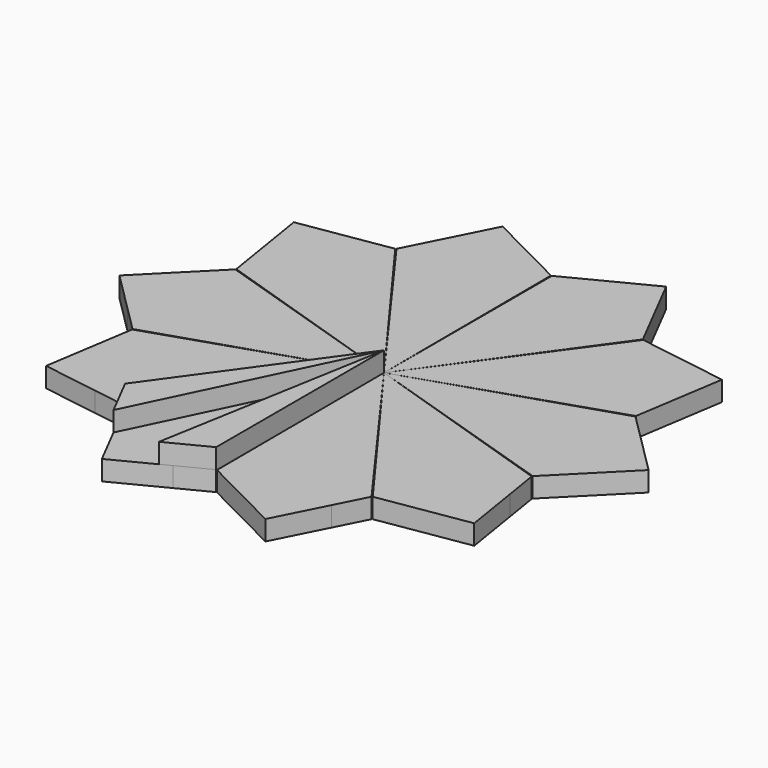
from build123d import *

# Parameters (mm, degrees)
F1_DEPTH = 10
F3_DEPTH = 10
F4_COUNT = 10


# Not quite as in the source:
# - a feature names something its author has since deleted; it is built from what else it names


with BuildPart() as f1:
    # F0 (on Top) → F1 (new body)
    with BuildSketch(Plane.XY):
        Polygon((-305.3184055859, -77.3749127087), (-289.8050833034, 36.5739215625), (-343.7715783939, -64.9771365691), (-330.7438800597, -90.4026110429), align=None)
        Polygon((-343.7715783939, -64.9771365691), (-289.8050833034, 36.5739215625), (-351.7204126651, -49.4638142865), align=None)
        Polygon((-289.8050833034, -69.4260784375), (-289.8050833034, 36.5739215625), (-305.3184055859, -77.3749127087), align=None)
    extrude(amount=F1_DEPTH)


with BuildPart() as f3:
    # F2 (on face) → F3 (new body)
    with BuildSketch(Plane.XY.offset(10)):
        Polygon((-289.8050833034, -69.4260784375), (-289.8050833034, 36.5739215625), (-310.2744816815, -79.9143447402), align=None)
    extrude(amount=F3_DEPTH)


with BuildPart() as f3b:
    # F2 (on face) → F3, piece 2 (new body)
    with BuildSketch(Plane.XY.offset(10)):
        Polygon((-341.2321463624, -69.9332126647), (-289.8050833034, 36.5739215625), (-351.7204126651, -49.4638142865), align=None)
    extrude(amount=F3_DEPTH)


with BuildPart() as f4_1:
    # F4: instance of F1
    add(f1.part.rotate(Axis((-289.8050833034, 36.5739215625, 5), (0, 0, -1)), 1 * 360 / F4_COUNT))


with BuildPart() as f4_2:
    # F4: instance of F1
    add(f1.part.rotate(Axis((-289.8050833034, 36.5739215625, 5), (0, 0, -1)), 2 * 360 / F4_COUNT))


with BuildPart() as f4_3:
    # F4: instance of F1
    add(f1.part.rotate(Axis((-289.8050833034, 36.5739215625, 5), (0, 0, -1)), 3 * 360 / F4_COUNT))


with BuildPart() as f4_4:
    # F4: instance of F1
    add(f1.part.rotate(Axis((-289.8050833034, 36.5739215625, 5), (0, 0, -1)), 4 * 360 / F4_COUNT))


with BuildPart() as f4_5:
    # F4: instance of F1
    add(f1.part.rotate(Axis((-289.8050833034, 36.5739215625, 5), (0, 0, -1)), 5 * 360 / F4_COUNT))


with BuildPart() as f4_6:
    # F4: instance of F1
    add(f1.part.rotate(Axis((-289.8050833034, 36.5739215625, 5), (0, 0, -1)), 6 * 360 / F4_COUNT))


with BuildPart() as f4_7:
    # F4: instance of F1
    add(f1.part.rotate(Axis((-289.8050833034, 36.5739215625, 5), (0, 0, -1)), 7 * 360 / F4_COUNT))


with BuildPart() as f4_8:
    # F4: instance of F1
    add(f1.part.rotate(Axis((-289.8050833034, 36.5739215625, 5), (0, 0, -1)), 8 * 360 / F4_COUNT))


with BuildPart() as f4_9:
    # F4: instance of F1
    add(f1.part.rotate(Axis((-289.8050833034, 36.5739215625, 5), (0, 0, -1)), 9 * 360 / F4_COUNT))


solid = Compound([f1.part, f3.part, f3b.part, f4_1.part, f4_2.part, f4_3.part, f4_4.part, f4_5.part, f4_6.part, f4_7.part, f4_8.part, f4_9.part])
